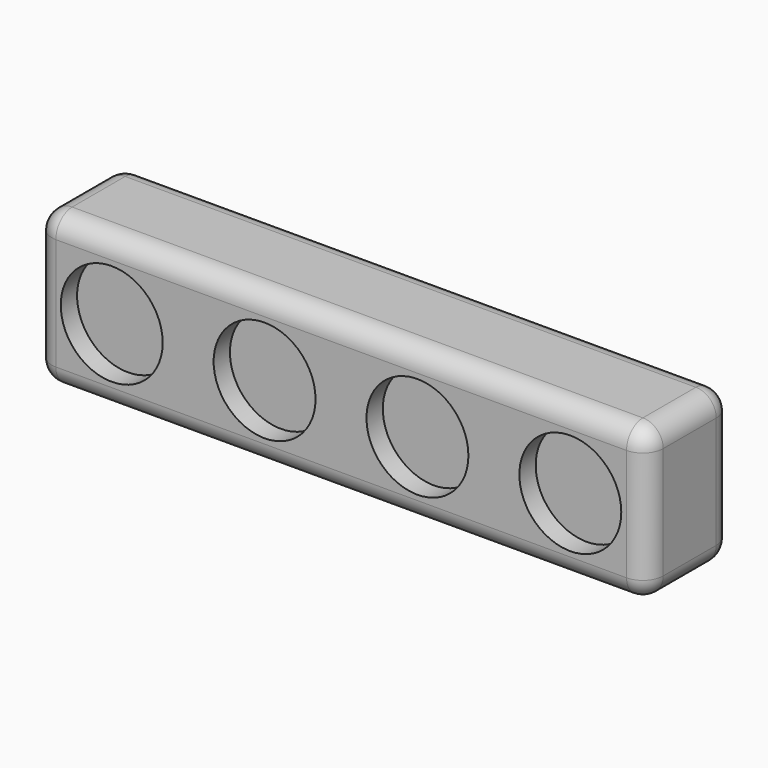
from build123d import *

# Parameters (mm, degrees)
F0_W     = 60
F0_H     = 15
F1_DEPTH = 10.5
F2_R     = 5
F3_DEPTH = 2
F4_R     = 2


# Not quite as in the source:
# - a feature names something its author has since deleted; it is built from what else it names


with BuildPart() as f1:
    # F0 (on Front) → F1 (new body)
    with BuildSketch(Plane.XZ):
        Rectangle(F0_W, F0_H)
    extrude(amount=F1_DEPTH)

    # F2 (on face) → F3 (cut)
    with BuildSketch(Plane.XZ.offset(10.5)):
        with Locations((-22.5179158151, 0)):
            Circle(F2_R)
        with Locations((-7.5179158151, 0)):
            Circle(F2_R)
        with Locations((7.4820841849, 0)):
            Circle(F2_R)
        with Locations((22.4820841849, 0)):
            Circle(F2_R)
    extrude(amount=-F3_DEPTH, mode=Mode.SUBTRACT)

    # F4
    f4_edges = [f1.edges().sort_by_distance(p)[0] for p in [
        (-30, -5.25, 7.5),
        (30, 0, 0),
        (0, -10.5, 7.5),
        (0, 0, 7.5),
        (30, -5.25, 7.5),
        (30, -5.25, -7.5),
        (30, -10.5, 0),
        (0, 0, -7.5),
        (-30, 0, 0),
        (-30, -5.25, -7.5),
        (-30, -10.5, 0),
        (0, -10.5, -7.5),
    ]]
    fillet(f4_edges, radius=F4_R)


solid = f1.part
